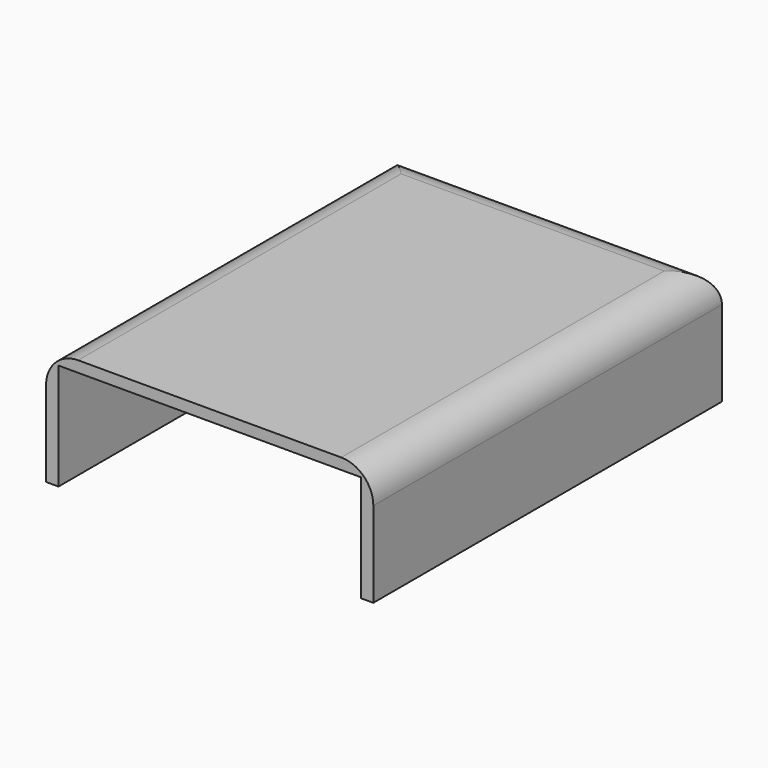
from build123d import *

# Parameters (mm, degrees)
F1_DEPTH    = 34.52499953
F2_T1_DEPTH = 94.44999906
F2_T3_DEPTH = 77.25000044


# Not quite as in the source:
# - a fillet or chamfer that OpenCascade refuses, or shapes differently, is made with other operations: its cross-section is extruded or revolved along the edge and cut away or added


with BuildPart() as f1:
    # F0 (on Front) → F1 (new body, symmetric)
    with BuildSketch(Plane.XZ):
        Polygon((21.5802040493, 18.630000078), (-30.2697963907, 18.630000078), (-30.2697963907, 0), (-28.3029927087, 0), (-28.3029927087, 16.8817297936), (19.6134003673, 16.8817297936), (19.6134003673, 0), (21.5802040493, 0), align=None)
    extrude(amount=F1_DEPTH, both=True)

    # F2: fillet of radius 5.08 on 3 edges, made by hand

    # F2_s2 → F2_t1 (cut)
    with BuildSketch(Plane.XZ.offset(-47.22499953)):
        with BuildLine():
            ThreePointArc((-25.1897963907, 18.630000078), (-28.7818988391, 17.1421025264), (-30.2697963907, 13.550000078))
            Line((-30.2697963907, 13.550000078), (-30.2697963907, 18.630000078))
            Line((-30.2697963907, 18.630000078), (-25.1897963907, 18.630000078))
        make_face()
        with BuildLine():
            ThreePointArc((16.5002040493, 18.630000078), (20.0923064978, 17.1421025264), (21.5802040493, 13.550000078))
            Line((21.5802040493, 13.550000078), (21.5802040493, 18.630000078))
            Line((21.5802040493, 18.630000078), (16.5002040493, 18.630000078))
        make_face()
    extrude(amount=F2_T1_DEPTH, mode=Mode.SUBTRACT)

    # F2_s4 → F2_t3 (cut)
    with BuildSketch(Plane.YZ.offset(-42.9697963907)):
        with BuildLine():
            ThreePointArc((29.44499953, 18.630000078), (33.0371019784, 17.1421025264), (34.52499953, 13.550000078))
            Line((34.52499953, 13.550000078), (34.52499953, 18.630000078))
            Line((34.52499953, 18.630000078), (29.44499953, 18.630000078))
        make_face()
    extrude(amount=F2_T3_DEPTH, mode=Mode.SUBTRACT)


solid = f1.part
